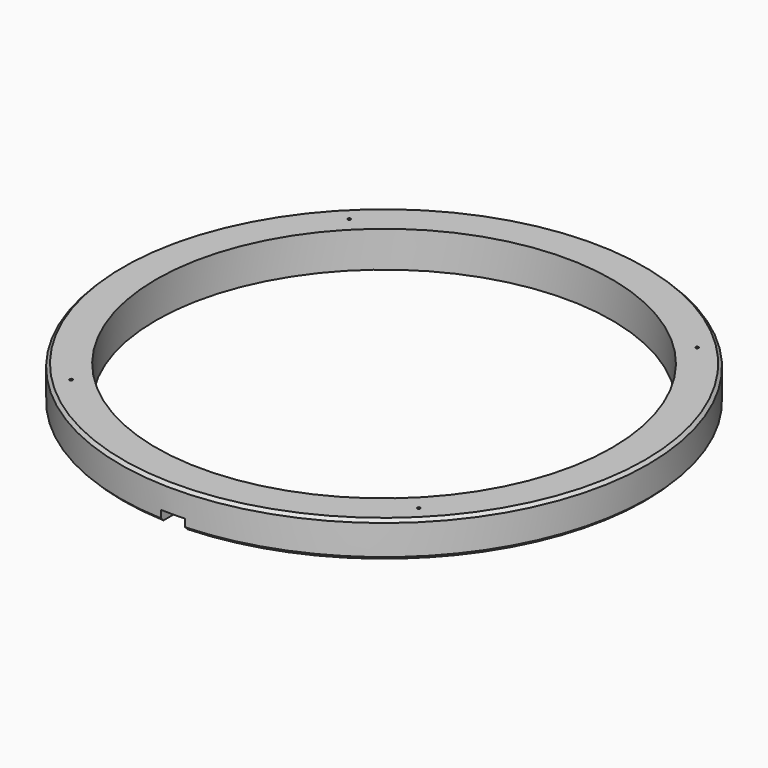
from build123d import *

# Parameters (mm, degrees)
F2_R      = 139.7
F3_DEPTH  = 19.05
F4_SIZE   = 1.5875
F5_R      = 120.65
F6_DEPTH  = 19.051
F7_W      = 12.7
F7_H      = 5.55625
F8_DEPTH  = 139.701
F9_R      = 0.79375
F10_DEPTH = 19.051


# Not quite as in the source:
# - a variable given as a bare number and used for a length is read in inches; the dataset says mm whatever the document's units were


with BuildPart() as f3:
    # F2 (on Top) → F3 (new body)
    with BuildSketch(Plane.XY):
        Circle(F2_R)
    extrude(amount=F3_DEPTH)

    # F4
    f4_edges = [f3.edges().sort_by_distance(p)[0] for p in [
        (-139.7, 0, 19.05),
        (-139.7, 0, 0),
    ]]
    chamfer(f4_edges, length=F4_SIZE)

    # F5 (on face) → F6 (cut, through all)
    with BuildSketch(Plane(origin=(0, 0, 0), x_dir=(1, 0, 0), z_dir=(0, 0, -1))):
        Circle(F5_R)
    extrude(amount=-F6_DEPTH, mode=Mode.SUBTRACT)

    # F7 (on Front) → F8 (cut, through all)
    with BuildSketch(Plane.XZ):
        with Locations((0, 2.778125)):
            Rectangle(F7_W, F7_H)
    extrude(amount=F8_DEPTH, mode=Mode.SUBTRACT)

    # F9 (on Top) → F10 (cut, through all)
    with BuildSketch(Plane.XY):
        with Locations((92.047625241, -92.047625241)):
            Circle(F9_R)
        with Locations((-92.047625241, -92.047625241)):
            Circle(F9_R)
        with Locations((-92.047625241, 92.047625241)):
            Circle(F9_R)
        with Locations((92.047625241, 92.047625241)):
            Circle(F9_R)
    extrude(amount=F10_DEPTH, mode=Mode.SUBTRACT)


solid = f3.part
